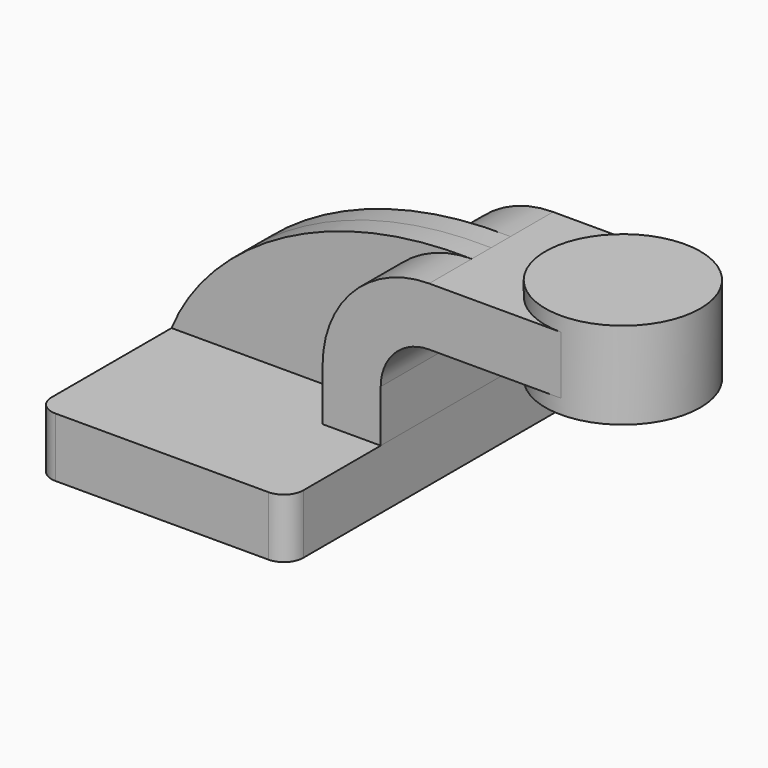
from build123d import *

# Parameters (mm, degrees)
F1_DEPTH = 63.5
F0_W     = 25.4
F0_H     = 19.05
F2_DEPTH = 25.4
F3_DEPTH = 7.9375
F5_R     = 6.35


with BuildPart() as f1:
    # F0 (on Front) → F1 (new body, symmetric)
    with BuildSketch(Plane.XZ):
        Polygon((22.225, 9.7409027457), (-41.275, 9.7409027457), (-41.275, -9.7409027457), (41.275, -9.7409027457), (41.275, 9.7409027457), align=None)
    extrude(amount=F1_DEPTH, both=True)

    # F0 (on Front) → F3 (join, symmetric)
    with BuildSketch(Plane.XZ):
        with BuildLine():
            add(Edge.make_bspline(
                [(-41.275, 9.7409027457), (-30.1918908954, 37.2608341277), (6.4949910156, 62.8735125065), (57.15, 61.7092972543)],
                knots=[0, 0, 0, 0, 111.3022670605, 111.3022670605, 111.3022670605, 111.3022670605], degree=3))
            Line((-41.275, 9.7409027457), (22.225, 9.7409027457))
            Line((22.225, 9.7409027457), (22.225, 26.7842972543))
            ThreePointArc((22.225, 26.7842972543), (32.4542956671, 51.4800015873), (57.15, 61.7092972543))
        make_face()
    extrude(amount=F3_DEPTH, both=True)

    # F5
    f5_edges = [f1.edges().sort_by_distance(p)[0] for p in [
        (-41.275, -63.5, 0),
        (41.275, -63.5, 0),
        (41.275, 63.5, 0),
        (-41.275, 63.5, 0),
    ]]
    fillet(f5_edges, radius=F5_R)


with BuildPart() as f2:
    # F0 (on Front) → F2 (new body, symmetric)
    with BuildSketch(Plane.XZ):
        with BuildLine():
            Line((22.225, 26.7842972543), (22.225, 9.7409027457))
            Line((22.225, 9.7409027457), (41.275, 9.7409027457))
            Line((41.275, 9.7409027457), (41.275, 26.7842972543))
            ThreePointArc((41.275, 26.7842972543), (45.9246798487, 38.0096174057), (57.15, 42.6592972543))
            Line((57.15, 42.6592972543), (74.9554038295, 42.6592972543))
            Line((74.9554038295, 42.6592972543), (74.9554038295, 61.7092972543))
            Line((74.9554038295, 61.7092972543), (57.15, 61.7092972543))
            ThreePointArc((57.15, 61.7092972543), (32.4542956671, 51.4800015873), (22.225, 26.7842972543))
        make_face()
        with Locations((87.6554038295, 52.1842972543)):
            Rectangle(F0_W, F0_H)
    extrude(amount=F2_DEPTH, both=True)

    # F0 (on Front) → F4 (revolve)
    with BuildSketch(Plane.XZ):
        Polygon((100.3554038295, 66.4590972543), (100.3554038295, 61.7092972543), (100.3554038295, 42.6592972543), (100.3554038295, 37.8840972543), (125.7554038295, 37.8840972543), (125.7554038295, 66.4590972543), align=None)
    revolve(axis=Axis((100.3554038295, 0, 52.1715972543), (0, 0, 1)))


solid = Compound([f1.part, f2.part])
